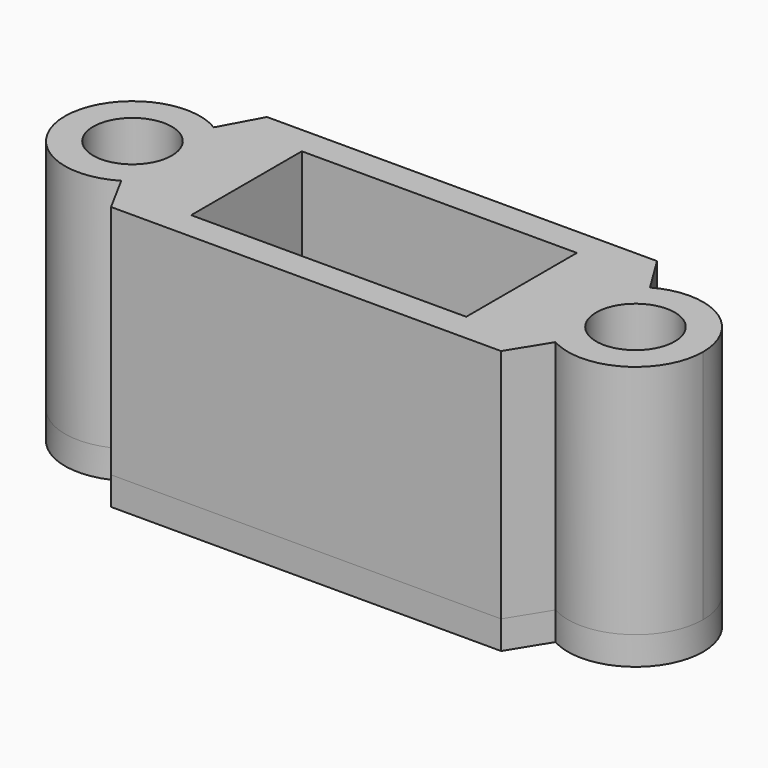
from build123d import *
from build123d import SkipClean  # not in build123d's __all__

# Parameters (mm, degrees)
F2_R     = 2.5
F2_W     = 17.5
F2_H     = 8.8
F3_DEPTH = 15
F4_R     = 2.5
F4_W     = 17.5
F4_H     = 8.8
F5_DEPTH = 1.8


with BuildPart() as f3:
    # F2 (on Top) → F3 (new body)
    with BuildSketch(Plane.XY):
        with BuildLine():
            ThreePointArc((-13.7742425586, -3.6791308501), (-12.2542853153, -2.1117815941), (-11.7, 0))
            ThreePointArc((-11.7, 0), (-12.2542853153, 2.1117815941), (-13.7742425586, 3.6791308501))
            ThreePointArc((-13.7742425586, 3.6791308501), (-20.3, 0), (-13.7742425586, -3.6791308501))
        make_face()
        with Locations((-16, 0)):
            Circle(F2_R, mode=Mode.SUBTRACT)
        with BuildLine():
            ThreePointArc((-13.7742425586, 3.6791308501), (-12.2542853153, 2.1117815941), (-11.7, 0))
            ThreePointArc((-11.7, 0), (-12.2542853153, -2.1117815941), (-13.7742425586, -3.6791308501))
            Line((-13.7742425586, -3.6791308501), (-12.4064937305, -6.2))
            Line((-12.4064937305, -6.2), (0, -6.2))
            Line((0, -6.2), (12.4064937305, -6.2))
            Line((12.4064937305, -6.2), (13.913982062, -3.7601235568))
            ThreePointArc((13.913982062, -3.7601235568), (11.7, 0), (13.913982062, 3.7601235568))
            Line((13.913982062, 3.7601235568), (12.4064937305, 6.2))
            Line((12.4064937305, 6.2), (0, 6.2))
            Line((0, 6.2), (-12.4064937305, 6.2))
            Line((-12.4064937305, 6.2), (-13.7742425586, 3.6791308501))
        make_face()
        Rectangle(F2_W, F2_H, mode=Mode.SUBTRACT)
        with BuildLine():
            ThreePointArc((20.3, 0), (18.1817565019, 3.705393173), (13.913982062, 3.7601235568))
            ThreePointArc((13.913982062, 3.7601235568), (11.7, 0), (13.913982062, -3.7601235568))
            ThreePointArc((13.913982062, -3.7601235568), (18.1817565019, -3.705393173), (20.3, 0))
        make_face()
        with Locations((16, 0)):
            Circle(F2_R, mode=Mode.SUBTRACT)
    extrude(amount=F3_DEPTH)

    # F4 (on face) → F5 (join)
    with BuildSketch(Plane(origin=(0, 0, 0), x_dir=(1, 0, 0), z_dir=(0, 0, -1))):
        with BuildLine():
            Line((-12.4064937305, 6.2), (-13.7742425586, 3.6791308501))
            ThreePointArc((-13.7742425586, 3.6791308501), (-20.3, 0), (-13.7742425586, -3.6791308501))
            Line((-13.7742425586, -3.6791308501), (-12.4064937305, -6.2))
            Line((-12.4064937305, -6.2), (12.4064937305, -6.2))
            Line((12.4064937305, -6.2), (13.913982062, -3.7601235568))
            ThreePointArc((13.913982062, -3.7601235568), (20.3, 0), (13.913982062, 3.7601235568))
            Line((13.913982062, 3.7601235568), (12.4064937305, 6.2))
            Line((12.4064937305, 6.2), (-12.4064937305, 6.2))
        make_face()
        with Locations((-16, 0)):
            Circle(F4_R, mode=Mode.SUBTRACT)
        Rectangle(F4_W, F4_H, mode=Mode.SUBTRACT)
        with Locations((16, 0)):
            Circle(F4_R, mode=Mode.SUBTRACT)
        Rectangle(F4_W, F4_H)
    with SkipClean():  # cleaning this boolean's faces spoils the solid; the shape is the same uncleaned
        extrude(amount=F5_DEPTH)


solid = f3.part
